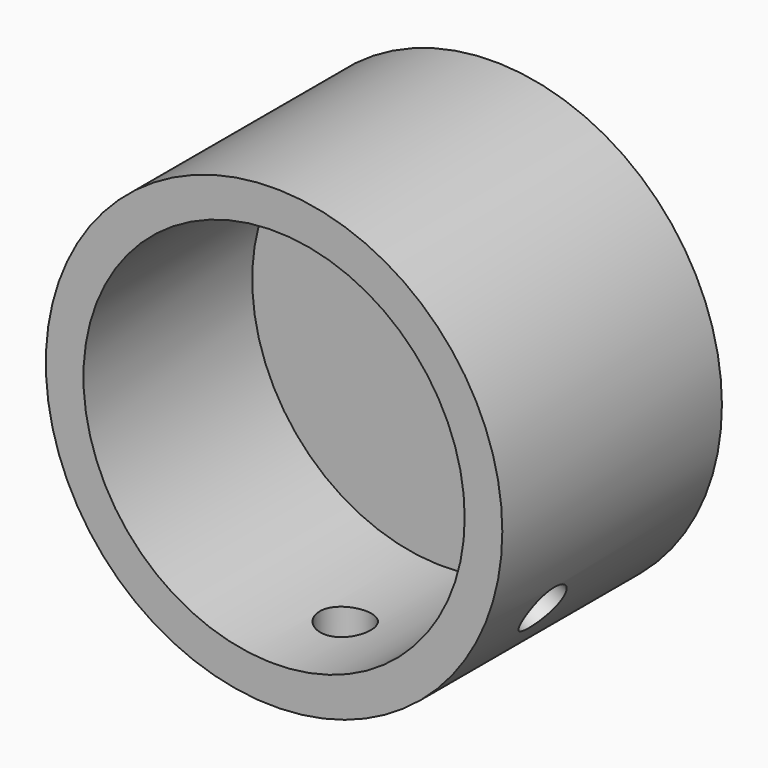
from build123d import *

# Parameters (mm, degrees)
F0_R      = 22.8092
F1_DEPTH  = 27.432
F3_DEPTH  = 14.986
F4_R      = 19.05
F5_DEPTH  = 21.082
F8_D      = 5.1054
F8_DEPTH  = 7.5692
F8_START  = 0.1432934
F8_TIP    = 1.5338169022
F12_D     = 5.1054
F12_DEPTH = 3.7592
F12_START = 0.1432934
F12_TIP   = 1.5338169022


with BuildPart() as f1:
    # F0 (on Front) → F1 (new body)
    with BuildSketch(Plane.XZ):
        Circle(F0_R)
    extrude(amount=F1_DEPTH)

    # F2 (on face) → F3 (join)
    with BuildSketch(Plane(origin=(0, 0, 0), x_dir=(-1, 0, 0), z_dir=(0, 1, 0))):
        with BuildLine():
            Line((0, -4.0005), (2.5840677236, -4.0005))
            ThreePointArc((2.5840677236, -4.0005), (0, 4.7625), (-2.5840677236, -4.0005))
            Line((-2.5840677236, -4.0005), (0, -4.0005))
        make_face()
    extrude(amount=F3_DEPTH)

    # F4 (on face) → F5 (cut)
    with BuildSketch(Plane.XZ.offset(27.432)):
        Circle(F4_R)
    extrude(amount=-F5_DEPTH, mode=Mode.SUBTRACT)

    # F8
    # its depths count from where the whole tool has entered the part; down to there all is cleared
    with Locations(Plane(origin=(0, 0, -22.8092), x_dir=(1, 0, 0), z_dir=(0, 0, -1)).offset(-F8_START)):
        with Locations((0, 18.542)):
            Hole(F8_D / 2, depth=F8_DEPTH)
            with Locations((0, 0, -(F8_DEPTH + F8_TIP / 2))):  # 118° drill point
                Cone(0, F8_D / 2, F8_TIP, mode=Mode.SUBTRACT)

    # F12
    # its depths count from where the whole tool has entered the part; down to there all is cleared
    with Locations(Plane(origin=(19.75334664, 0, -11.4046), x_dir=(0, 1, 0), z_dir=(0.8660254038, 0, -0.5)).offset(-F12_START)):
        with Locations((-18.542, 0)):
            Hole(F12_D / 2, depth=F12_DEPTH)
            with Locations((0, 0, -(F12_DEPTH + F12_TIP / 2))):  # 118° drill point
                Cone(0, F12_D / 2, F12_TIP, mode=Mode.SUBTRACT)


solid = f1.part
